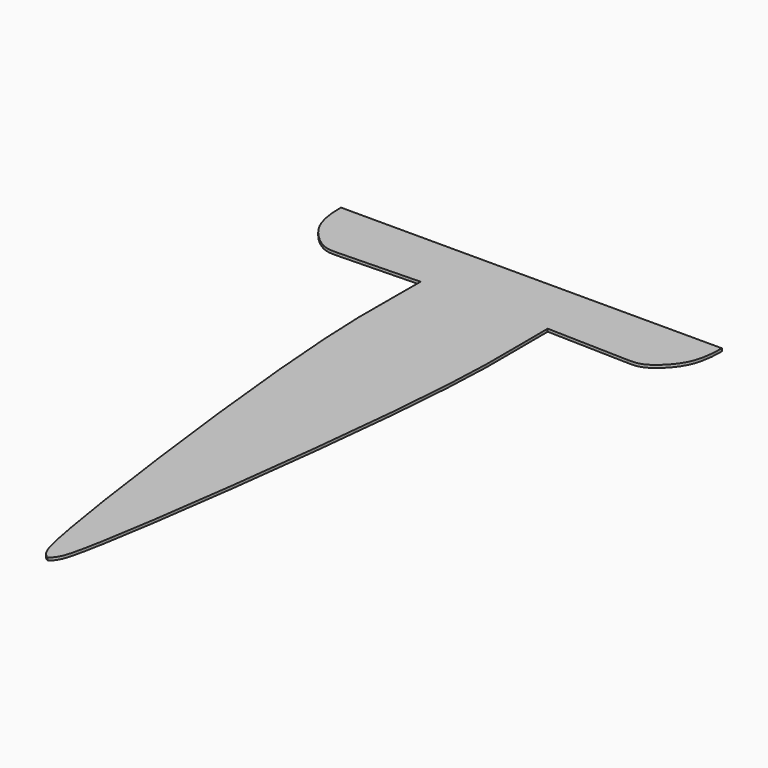
from build123d import *

# Parameters (mm, degrees)
F1_DEPTH = 10


with BuildPart() as f1:
    # F0 (on Top) → F1 (new body)
    with BuildSketch(Plane.XY):
        with BuildLine():
            Line((0, 85.2085053921), (0, -2128.7469863892))
            add(Edge.make_bspline(
                [(0, -2128.7469863892), (23.4590560131, -2115.0394865653), (59.9170876984, -2011.671111051), (178.1400323392, -1163.3441643463), (243.8064615583, -449.7847110684), (230.7232242509, -219.4097479535), (232.4981689453, -130.9822052717)],
                knots=[0, 0, 0, 0, 0.1206653396, 0.4678392709, 0.7964320829, 1, 1, 1, 1], degree=3))
            Line((232.4981689453, -130.9822052717), (531.4212441444, -139.2431110144))
            add(Edge.make_bspline(
                [(697.026848793, 85.2085053921), (697.5812315941, 54.1675575078), (692.2096198324, -0.9683446135), (663.0294773679, -71.7880519639), (586.4163084622, -141.5486278427), (548.5482408364, -138.9749926828), (531.4212441444, -139.2431110144)],
                knots=[0, 0, 0, 0, 0.2640358398, 0.5142505251, 0.7944573855, 1, 1, 1, 1], degree=3))
            Line((697.026848793, 85.2085053921), (0, 85.2085053921))
        make_face()
    extrude(amount=-F1_DEPTH)

    # F2: F1 across plane


with BuildPart() as f1_1:
    add(f1.part)
    add(f1.part.mirror(Plane.YZ))


solid = f1_1.part
